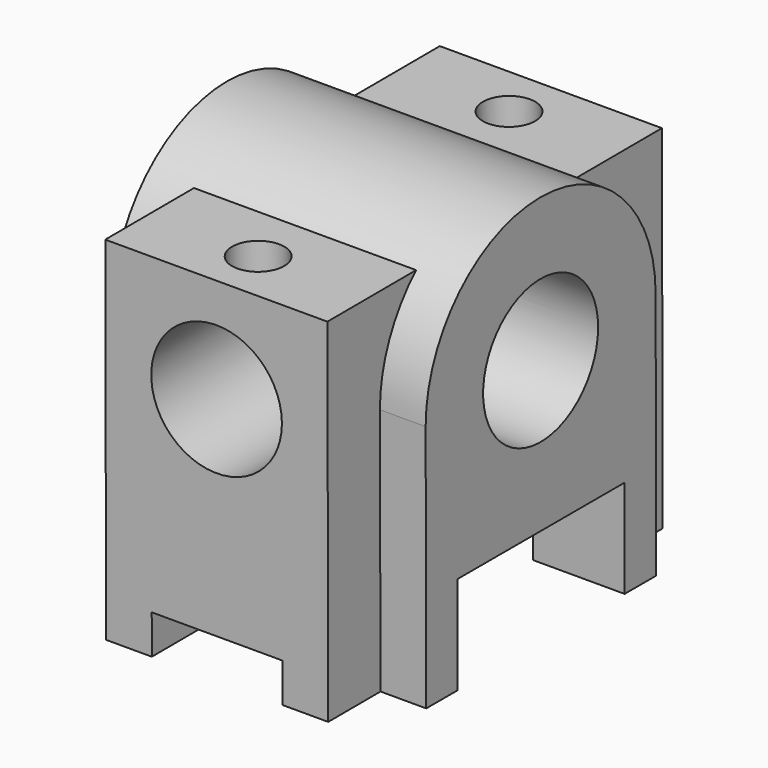
from build123d import *

# Parameters (mm, degrees)
F0_R      = 11
F1_DEPTH  = 24
F3_R      = 10
F6_R      = 10
F8_R      = 4
F9_DEPTH  = 5
F10_R     = 10
F11_DEPTH = 64.178337


with BuildPart() as f1:
    # F0 (on Right) → F1 (new body, symmetric)
    with BuildSketch(Plane.YZ):
        with BuildLine():
            Line((23.519836, -52.259333), (29.564144, -52.259333))
            Line((29.564144, -52.259333), (29.451314, -14.144763))
            ThreePointArc((29.451314, -14.144763), (7.400617, 7.740608), (-14.548384, -14.246754))
            Line((-14.548384, -14.246754), (-14.435856, -52.259333))
            Line((-14.435856, -52.259333), (-8.480164, -52.259333))
            Line((-8.480164, -52.259333), (-8.480164, -37.259333))
            Line((-8.480164, -37.259333), (23.519836, -37.259333))
            Line((23.519836, -37.259333), (23.519836, -52.259333))
        make_face()
        with Locations((7.451612, -14.259333)):
            Circle(F0_R, mode=Mode.SUBTRACT)
    extrude(amount=F1_DEPTH, both=True)

    # F3 (on offset) → F4 (join, up to the next surface of F1)
    with BuildSketch(Plane(origin=(0, -24.590387, -0.072795), x_dir=(1, 0, 0), z_dir=(0, -0.999996, -0.00296))):
        Polygon((-10, -52.21637), (-10, -46.21637), (10, -46.21637), (10, -52.21637), (17, -52.21637), (17, 1.78363), (-17, 1.78363), (-17, -52.21637), align=None)
        with Locations((0, -14.21637)):
            Circle(F3_R, mode=Mode.SUBTRACT)
    extrude(until=Until.NEXT, dir=(0, 0.999996, 0.00296))

    # F6 (on offset) → F7 (join, up to the next surface of F1)
    with BuildSketch(Plane(origin=(0, 39.409139, 0.116663), x_dir=(-1, 0, 0), z_dir=(0, 0.999996, 0.00296))):
        Polygon((-17, 1.653377), (-17, -52.346623), (-10, -52.346623), (-10, -46.346623), (10, -46.346623), (10, -52.346623), (17, -52.346623), (17, 1.653377), align=None)
        with Locations((0, -14.346623)):
            Circle(F6_R, mode=Mode.SUBTRACT)
    extrude(until=Until.NEXT, dir=(0, -0.999996, -0.00296))

    # F8 (on face) → F9 (cut)
    with BuildSketch(Plane(origin=(0, -0.00528, 1.783622), x_dir=(1, 0, 0), z_dir=(0, -0.00296, 0.999996))):
        with Locations((0, -16.590688)):
            Circle(F8_R)
        with Locations((0, 31.409312)):
            Circle(F8_R)
    extrude(amount=-F9_DEPTH, mode=Mode.SUBTRACT)

    # F10 (on face) → F11 (cut, through all)
    with BuildSketch(Plane(origin=(0, -24.590387, -0.072795), x_dir=(1, 0, 0), z_dir=(0, -0.999996, -0.00296))):
        with Locations((0, -14.21637)):
            Circle(F10_R)
        Polygon((10, -46.21637), (-10, -46.21637), (-10, -52.21637), (-10, -63.314267), (10, -63.314267), (10, -52.21637), align=None)
    extrude(amount=-F11_DEPTH, mode=Mode.SUBTRACT)


solid = f1.part
